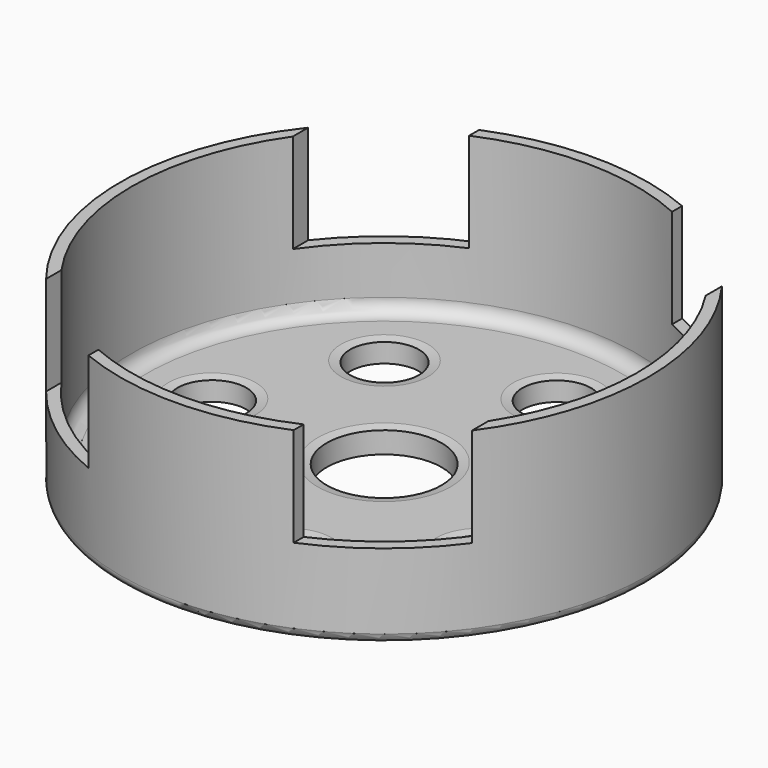
from build123d import *

# Parameters (mm, degrees)
F0_R           = 57.5
F1_DEPTH       = 40
F2_R           = 55
F3_DEPTH       = 35
F4_R           = 3
F5_R           = 2
F6_R           = 12.5
F7_DEPTH       = 40.001
F9_D           = 15
F9_CBORE_D     = 20
F9_CBORE_DEPTH = 0.5
F10_C1_SIZE2   = 2
F10_C1_SIZE    = 0.3526539614
F10_C2_SIZE2   = 0.3526539614
F10_C2_SIZE    = 2
F10_C3_SIZE2   = 0.3526539614
F10_C3_SIZE    = 2
F10_C4_SIZE2   = 0.3526539614
F10_C4_SIZE    = 2
F10_C5_SIZE2   = 0.3526539614
F10_C5_SIZE    = 2
F10_C6_SIZE2   = 0.3526539614
F10_C6_SIZE    = 2
F10_C7_SIZE2   = 0.3526539614
F10_C7_SIZE    = 2
F10_C8_SIZE2   = 0.3526539614
F10_C8_SIZE    = 2
F11_W          = 23.2258066535
F11_H          = 27.9435478151
F11_W_2        = 23.7701628357
F11_H_2        = 28.1250029802
F12_DEPTH      = 57.5010001
F12_DEPTH_BACK = 57.5010001


with BuildPart() as f1:
    # F0 (on Top) → F1 (new body)
    with BuildSketch(Plane.XY):
        Circle(F0_R)
    extrude(amount=F1_DEPTH)

    # F2 (on face) → F3 (cut)
    with BuildSketch(Plane.XY.offset(40)):
        Circle(F2_R)
    extrude(amount=-F3_DEPTH, mode=Mode.SUBTRACT)

    # F4
    f4_edges = [f1.edges().sort_by_distance(p)[0] for p in [
        (-55, 0, 5),
    ]]
    fillet(f4_edges, radius=F4_R)

    # F5
    f5_edges = [f1.edges().sort_by_distance(p)[0] for p in [
        (-57.5, 0, 0),
    ]]
    fillet(f5_edges, radius=F5_R)

    # F6 (on face) → F7 (cut, through all)
    with BuildSketch(Plane(origin=(0, 0, 0), x_dir=(1, 0, 0), z_dir=(0, 0, -1))):
        Circle(F6_R)
    extrude(amount=-F7_DEPTH, mode=Mode.SUBTRACT)

    # F9 (through all)
    with Locations(Plane(origin=(0, 0, 0), x_dir=(1, 0, 0), z_dir=(0, 0, -1))):
        with Locations((-37.5, 0), (-23.3808675697, 29.3186805926), (8.3445350234, 36.5597967068), (33.7863325463, 16.2706402169), (33.7863325463, -16.2706402169), (8.3445350234, -36.5597967068), (-23.3808675697, -29.3186805926)):
            CounterBoreHole(F9_D / 2, F9_CBORE_D / 2, F9_CBORE_DEPTH)

    # F10: chamfer of 2 x 0.3526539614 on 8 edges, made by hand

    # F10_c1
    f10_c1_edges = [f1.edges().sort_by_distance(p)[0] for p in [
        (-12.5, 0, 5),
    ]]
    f10_c1_side = f1.faces().sort_by_distance((-12.5, 0, 4.9929469208))[0]
    chamfer(f10_c1_edges, length=F10_C1_SIZE, length2=F10_C1_SIZE2, reference=f10_c1_side)

    # F10_c2
    f10_c2_edges = [f1.edges().sort_by_distance(p)[0] for p in [
        (-30.8808675697, -29.3186805926, 5),
    ]]
    f10_c2_side = f1.faces().sort_by_distance((-30.8879206489, -29.3186805926, 5))[0]
    chamfer(f10_c2_edges, length=F10_C2_SIZE, length2=F10_C2_SIZE2, reference=f10_c2_side)

    # F10_c3
    f10_c3_edges = [f1.edges().sort_by_distance(p)[0] for p in [
        (0.8445350234, -36.5597967068, 5),
    ]]
    f10_c3_side = f1.faces().sort_by_distance((0.8374819441, -36.5597967068, 5))[0]
    chamfer(f10_c3_edges, length=F10_C3_SIZE, length2=F10_C3_SIZE2, reference=f10_c3_side)

    # F10_c4
    f10_c4_edges = [f1.edges().sort_by_distance(p)[0] for p in [
        (26.2863325463, -16.2706402169, 5),
    ]]
    f10_c4_side = f1.faces().sort_by_distance((26.2792794671, -16.2706402169, 5))[0]
    chamfer(f10_c4_edges, length=F10_C4_SIZE, length2=F10_C4_SIZE2, reference=f10_c4_side)

    # F10_c5
    f10_c5_edges = [f1.edges().sort_by_distance(p)[0] for p in [
        (-45, 0, 5),
    ]]
    f10_c5_side = f1.faces().sort_by_distance((-45.0070530792, 0, 5))[0]
    chamfer(f10_c5_edges, length=F10_C5_SIZE, length2=F10_C5_SIZE2, reference=f10_c5_side)

    # F10_c6
    f10_c6_edges = [f1.edges().sort_by_distance(p)[0] for p in [
        (-30.8808675697, 29.3186805926, 5),
    ]]
    f10_c6_side = f1.faces().sort_by_distance((-30.8879206489, 29.3186805926, 5))[0]
    chamfer(f10_c6_edges, length=F10_C6_SIZE, length2=F10_C6_SIZE2, reference=f10_c6_side)

    # F10_c7
    f10_c7_edges = [f1.edges().sort_by_distance(p)[0] for p in [
        (26.2863325463, 16.2706402169, 5),
    ]]
    f10_c7_side = f1.faces().sort_by_distance((26.2792794671, 16.2706402169, 5))[0]
    chamfer(f10_c7_edges, length=F10_C7_SIZE, length2=F10_C7_SIZE2, reference=f10_c7_side)

    # F10_c8
    f10_c8_edges = [f1.edges().sort_by_distance(p)[0] for p in [
        (0.8445350234, 36.5597967068, 5),
    ]]
    f10_c8_side = f1.faces().sort_by_distance((0.8374819441, 36.5597967068, 5))[0]
    chamfer(f10_c8_edges, length=F10_C8_SIZE, length2=F10_C8_SIZE2, reference=f10_c8_side)

    # F11 (on Front) → F12 (cut, two sides)
    with BuildSketch(Plane.XZ) as f12_sk:
        with Locations((-33.4778241813, 32.3891136795)):
            Rectangle(F11_W, F11_H)
        with Locations((34.4758061692, 32.4798412621)):
            Rectangle(F11_W_2, F11_H_2)
    extrude(amount=F12_DEPTH, mode=Mode.SUBTRACT)
    extrude(f12_sk.sketch, amount=-F12_DEPTH_BACK, mode=Mode.SUBTRACT)


solid = f1.part
